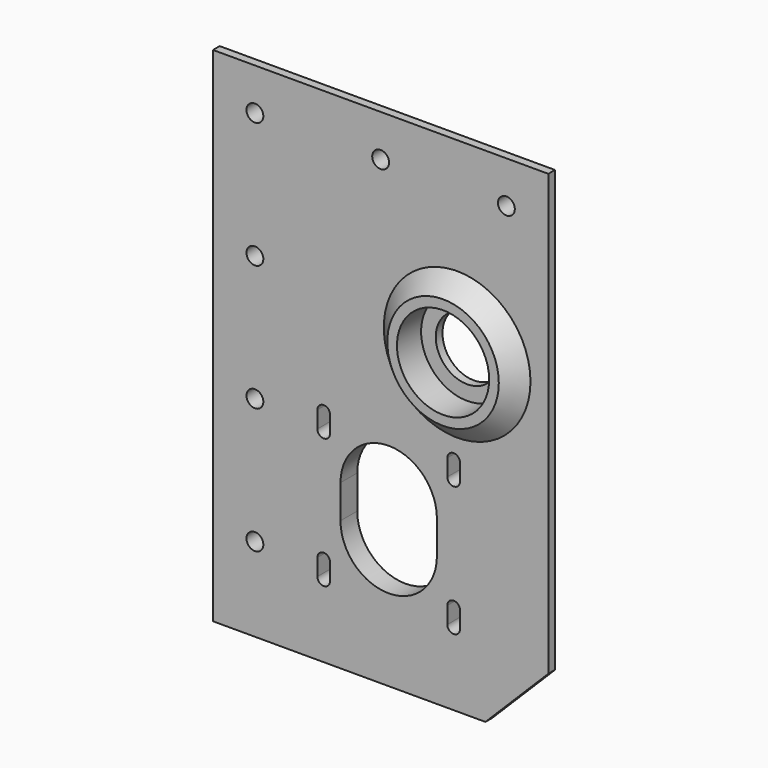
from build123d import *

# Parameters (mm, degrees)
F0_R     = 2.01
F0_R_2   = 7.5
F1_DEPTH = 5
F2_SIZE  = 3
F3_R     = 11
F4_DEPTH = 3
F5_R     = 17.5
F5_R_2   = 11
F6_DEPTH = 4.2
F7_SIZE  = 4.19999


# Not quite as in the source:
# - a fillet or chamfer is up to 0.001 mm smaller than in the source, because OpenCascade refuses the exact size


with BuildPart() as f1:
    # F0 (on Front) → F1 (new body)
    with BuildSketch(Plane.XZ):
        Polygon((0, 70), (0, 0), (0, -50), (65, -50), (80, -35), (80, 70), align=None)
        with Locations((10, -30)):
            Circle(F0_R, mode=Mode.SUBTRACT)
        with BuildLine():
            ThreePointArc((24.9080765748, -28.5), (26.4180765748, -26.99), (27.9280765748, -28.5))
            Line((27.9280765748, -28.5), (27.9280765748, -32.5))
            ThreePointArc((27.9280765748, -32.5), (26.4180765748, -34.01), (24.9080765748, -32.5))
            Line((24.9080765748, -32.5), (24.9080765748, -28.5))
        make_face(mode=Mode.SUBTRACT)
        with Locations((10, 0)):
            Circle(F0_R, mode=Mode.SUBTRACT)
        with BuildLine():
            ThreePointArc((27.9280765748, -1.5), (26.4180765748, -3.01), (24.9080765748, -1.5))
            Line((24.9080765748, -1.5), (24.9080765748, 2.5))
            ThreePointArc((24.9080765748, 2.5), (26.4180765748, 4.01), (27.9280765748, 2.5))
            Line((27.9280765748, 2.5), (27.9280765748, -1.5))
        make_face(mode=Mode.SUBTRACT)
        with BuildLine():
            ThreePointArc((55.9080765748, -28.5), (57.4180765748, -26.99), (58.9280765748, -28.5))
            Line((58.9280765748, -28.5), (58.9280765748, -32.5))
            ThreePointArc((58.9280765748, -32.5), (57.4180765748, -34.01), (55.9080765748, -32.5))
            Line((55.9080765748, -32.5), (55.9080765748, -28.5))
        make_face(mode=Mode.SUBTRACT)
        with BuildLine():
            ThreePointArc((30.4180765748, -11), (41.9180765748, 0.5), (53.4180765748, -11))
            Line((53.4180765748, -11), (53.4180765748, -19))
            ThreePointArc((53.4180765748, -19), (41.9180765748, -30.5), (30.4180765748, -19))
            Line((30.4180765748, -19), (30.4180765748, -11))
        make_face(mode=Mode.SUBTRACT)
        with BuildLine():
            ThreePointArc((58.9280765748, -1.5), (57.4180765748, -3.01), (55.9080765748, -1.5))
            Line((55.9080765748, -1.5), (55.9080765748, 2.5))
            ThreePointArc((55.9080765748, 2.5), (57.4180765748, 4.01), (58.9280765748, 2.5))
            Line((58.9280765748, 2.5), (58.9280765748, -1.5))
        make_face(mode=Mode.SUBTRACT)
        with Locations((10, 30)):
            Circle(F0_R, mode=Mode.SUBTRACT)
        with Locations((10, 60)):
            Circle(F0_R, mode=Mode.SUBTRACT)
        with Locations((58.25, 25)):
            Circle(F0_R_2, mode=Mode.SUBTRACT)
        with Locations((40, 60)):
            Circle(F0_R, mode=Mode.SUBTRACT)
        with Locations((70, 60)):
            Circle(F0_R, mode=Mode.SUBTRACT)
    extrude(amount=F1_DEPTH)

    # F2
    f2_edges = [f1.edges().sort_by_distance(p)[0] for p in [
        (80, 0, 17.5),
        (40, 0, 70),
        (0, 0, 10),
        (32.5, 0, -50),
        (72.5, 0, -42.5),
    ]]
    chamfer(f2_edges, length=F2_SIZE)

    # F3 (on face) → F4 (cut)
    with BuildSketch(Plane.XZ.offset(5)):
        with Locations((58.25, 25)):
            Circle(F3_R)
    extrude(amount=-F4_DEPTH, mode=Mode.SUBTRACT)

    # F5 (on face) → F6 (join)
    with BuildSketch(Plane.XZ.offset(5)):
        with Locations((58.25, 25)):
            Circle(F5_R)
        with Locations((58.25, 25)):
            Circle(F5_R_2, mode=Mode.SUBTRACT)
    extrude(amount=F6_DEPTH)

    # F7 (size 4.2 in the source; OpenCascade refuses exactly that, so slightly less here)
    f7_edges = [f1.edges().sort_by_distance(p)[0] for p in [
        (40.75, -9.2, 25),
    ]]
    chamfer(f7_edges, length=F7_SIZE)


solid = f1.part
